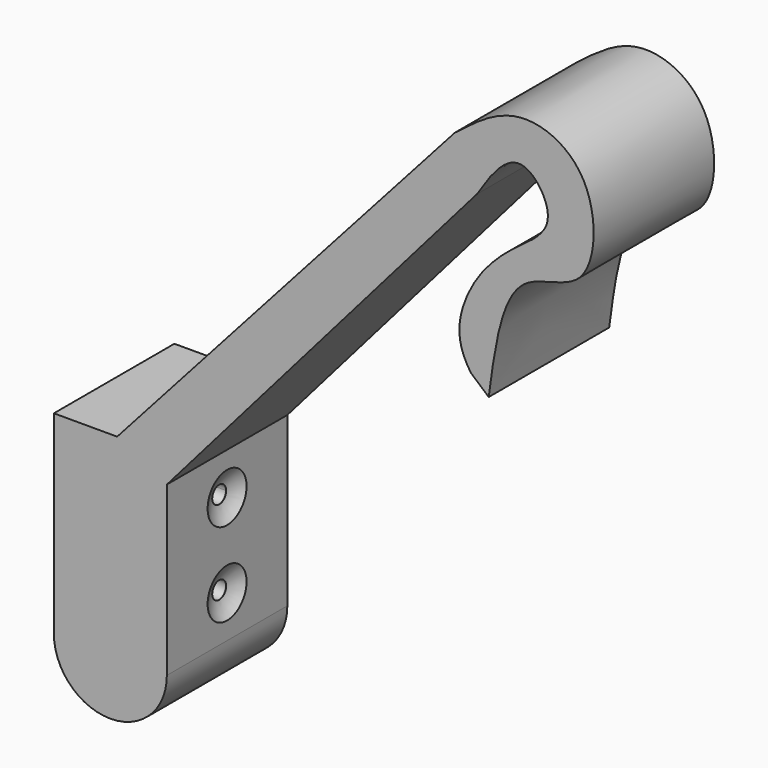
from build123d import *

# Parameters (mm, degrees)
F0_W      = 80
F0_H      = 100
F1_DEPTH  = 22
F3_DEPTH  = 25.4
F5_DEPTH  = 25.4
F7_DEPTH  = 1.27
F9_R      = 1.27
F10_DEPTH = 15.2322796478
F11_R     = 1.27
F12_DEPTH = 25.4
F13_R     = 1.27
F14_DEPTH = 25.4
F15_R     = 1.27
F16_DEPTH = 25.4


# Not quite as in the source:
# - a fillet or chamfer that OpenCascade refuses, or shapes differently, is made with other operations: its cross-section is extruded or revolved along the edge and cut away or added


with BuildPart() as f1:
    # F0 (on Front) → F1 (new body)
    with BuildSketch(Plane.XZ):
        with Locations((40, 50)):
            Rectangle(F0_W, F0_H)
    extrude(amount=F1_DEPTH)

    # F2 (on face) → F3 (cut)
    with BuildSketch(Plane.XZ.offset(22)):
        with BuildLine():
            Line((0, 100), (0, 36.83))
            Line((0, 36.83), (9.2459851876, 36.83))
            Line((9.2459851876, 36.83), (58.5819929838, 91.97023453))
            add(Edge.make_bspline(
                [(58.5819929838, 91.97023453), (61.6199278133, 94.3505869317), (67.6561205569, 99.0802031682), (79.6579791633, 93.6458192132), (79.1829808417, 76.6947426088), (65.9701540772, 78.137295591), (64.4170150326, 66.3796250164), (63.517652452, 59.5712140203)],
                knots=[0, 0, 0, 0, 0.191118588, 0.3797410737, 0.5865843575, 0.7606070362, 1, 1, 1, 1], degree=3))
            Line((63.517652452, 59.5712140203), (60.9292132491, 61.8223100773))
            add(Edge.make_bspline(
                [(61.8246197701, 85.1464193763), (64.9645352541, 90.2523029964), (68.8437089135, 93.0278581679), (74.1544737157, 84.3547705184), (66.7036385759, 79.9296548946), (61.5440518547, 74.6818576875), (58.6407715513, 67.8751926872), (59.4429238606, 63.9983425872), (60.9292132491, 61.8223100773)],
                knots=[0, 0, 0, 0, 0.1875888939, 0.3434475363, 0.5101787713, 0.6824698633, 0.8442602107, 1, 1, 1, 1], degree=3))
            Line((61.8246197701, 85.1464193763), (16.5012795478, 33.0310463905))
            Line((16.5012795478, 33.0310463905), (16.5012795478, 0))
            Line((16.5012795478, 0), (80, 0))
            Line((80, 0), (80, 100))
            Line((80, 100), (0, 100))
        make_face()
    extrude(amount=-F3_DEPTH, mode=Mode.SUBTRACT)

    # F4 (on face) → F5 (cut)
    with BuildSketch(Plane.XZ.offset(22)):
        with BuildLine():
            Line((16.5012795478, 0), (16.5012795478, 8.4898779529))
            ThreePointArc((16.5012795478, 8.4898779529), (8.2506397739, 0.239238179), (0, 8.4898779529))
            Line((0, 8.4898779529), (0, 0))
            Line((0, 0), (16.5012795478, 0))
        make_face()
    extrude(amount=-F5_DEPTH, mode=Mode.SUBTRACT)

    # F6 (on face) → F7 (cut)
    with BuildSketch(Plane.YZ.offset(16.5012795478)):
        with BuildLine():
            Line((-11, 23.3397542811), (-11, 30.4517542811))
            ThreePointArc((-11, 30.4517542811), (-14.556, 26.8957542811), (-11, 23.3397542811))
        make_face()
        with BuildLine():
            ThreePointArc((-7.444, 26.8957542811), (-8.4855282861, 29.410225995), (-11, 30.4517542811))
            Line((-11, 30.4517542811), (-11, 23.3397542811))
            ThreePointArc((-11, 23.3397542811), (-8.4855282861, 24.3812825672), (-7.444, 26.8957542811))
        make_face()
        with BuildLine():
            ThreePointArc((-11, 18.1811700623), (-14.556, 14.6251700623), (-11, 11.0691700623))
            Line((-11, 11.0691700623), (-11, 18.1811700623))
        make_face()
        with BuildLine():
            Line((-11, 18.1811700623), (-11, 11.0691700623))
            ThreePointArc((-11, 11.0691700623), (-8.4855282861, 12.1106983484), (-7.444, 14.6251700623))
            ThreePointArc((-7.444, 14.6251700623), (-8.4855282861, 17.1396417762), (-11, 18.1811700623))
        make_face()
    extrude(amount=-F7_DEPTH, mode=Mode.SUBTRACT)

    # F8: fillet of radius 5.08 on 2 edges, made by hand

    # F8_s1 → F8_t2 (revolve)
    with BuildSketch(Plane.XZ.offset(11)):
        with BuildLine():
            ThreePointArc((16.5012795478, 23.3397542811), (15.5593746666, 24.903807222), (15.2312795478, 26.6998584462))
            Line((15.2312795478, 26.6998584462), (15.2312795478, 23.3397542811))
            Line((15.2312795478, 23.3397542811), (16.5012795478, 23.3397542811))
        make_face()
    revolve(axis=Axis((15.2312795478, -11, 26.8957542811), (1, 0, 0)))

    # F8_s3 → F8_t4 (revolve)
    with BuildSketch(Plane.XZ.offset(11)):
        with BuildLine():
            ThreePointArc((16.5012795478, 11.0691700623), (15.5593746666, 12.6332230032), (15.2312795478, 14.4292742274))
            Line((15.2312795478, 14.4292742274), (15.2312795478, 11.0691700623))
            Line((15.2312795478, 11.0691700623), (16.5012795478, 11.0691700623))
        make_face()
    revolve(axis=Axis((15.2312795478, -11, 14.6251700623), (1, 0, 0)))

    # F9 (on face) → F10 (cut, through all)
    with BuildSketch(Plane.YZ.offset(15.2312795478)):
        with Locations((-11, 26.8957542811)):
            Circle(F9_R)
    extrude(amount=-F10_DEPTH, mode=Mode.SUBTRACT)

    # F11 (on face) → F12 (cut)
    with BuildSketch(Plane(origin=(0, 0, 0), x_dir=(0, -1, 0), z_dir=(-1, 0, 0))):
        with Locations((11, 26.8957542811)):
            Circle(F11_R)
    extrude(amount=-F12_DEPTH, mode=Mode.SUBTRACT)

    # F13 (on face) → F14 (cut)
    with BuildSketch(Plane.YZ.offset(15.2312795478)):
        with Locations((-11, 14.6251700623)):
            Circle(F13_R)
    extrude(amount=-F14_DEPTH, mode=Mode.SUBTRACT)

    # F15 (on face) → F16 (cut)
    with BuildSketch(Plane(origin=(15.2312795478, 0, 0), x_dir=(0, -1, 0), z_dir=(-1, 0, 0))):
        with Locations((11, 14.6251700623)):
            Circle(F15_R)
    extrude(amount=-F16_DEPTH, mode=Mode.SUBTRACT)


solid = f1.part
